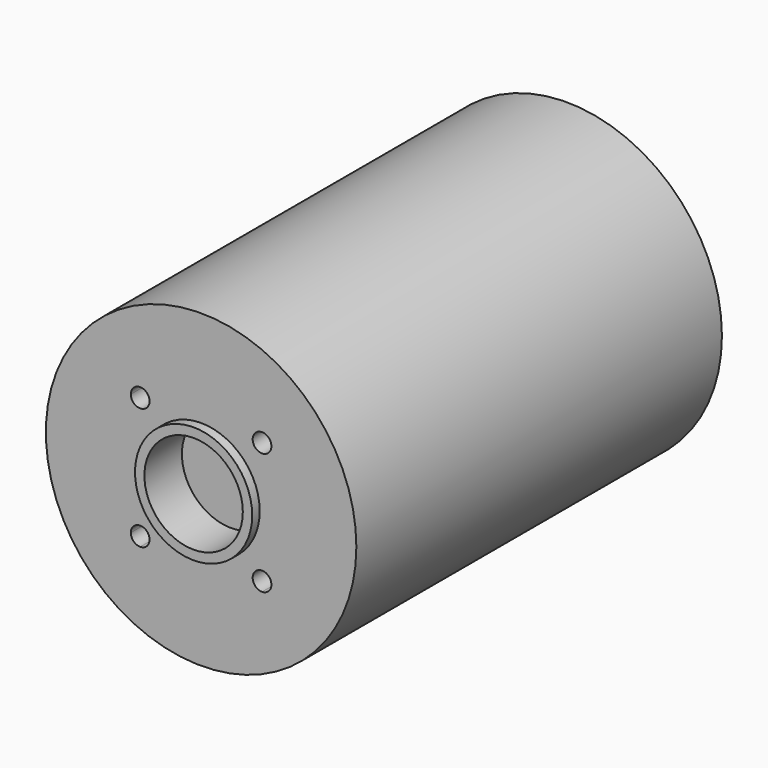
from build123d import *

# Parameters (mm, degrees)
F0_R     = 84.1375
F1_DEPTH = 247.65
F2_R     = 31.75
F3_DEPTH = 5.08
F5_DEPTH = 25.4
F6_R     = 26.67
F7_DEPTH = 25.4


# Not quite as in the source:
# - a feature names something its author has since deleted; it is built from what else it names


with BuildPart() as f1:
    # F0 (on Front) → F1 (new body)
    with BuildSketch(Plane.XZ):
        Circle(F0_R)
    extrude(amount=F1_DEPTH)

    # F2 (on face) → F3 (join)
    with BuildSketch(Plane.XZ.offset(247.65)):
        Circle(F2_R)
    extrude(amount=F3_DEPTH)

    # F4 (on face) → F5 (cut)
    with BuildSketch(Plane.XZ.offset(247.65)):
        with BuildLine():
            ThreePointArc((-27.94, 33.02), (-29.4278975516, 36.6121024484), (-33.02, 38.1))
            ThreePointArc((-33.02, 38.1), (-36.6121024484, 36.6121024484), (-38.1, 33.02))
            ThreePointArc((-38.1, 33.02), (-33.02, 27.94), (-27.94, 33.02))
        make_face()
        with BuildLine():
            ThreePointArc((38.1, 33.02), (36.6121024484, 36.6121024484), (33.02, 38.1))
            ThreePointArc((33.02, 38.1), (29.4278975516, 29.4278975516), (38.1, 33.02))
        make_face()
        with BuildLine():
            ThreePointArc((33.02, -38.1), (36.6121024484, -36.6121024484), (38.1, -33.02))
            ThreePointArc((38.1, -33.02), (29.4278975516, -29.4278975516), (33.02, -38.1))
        make_face()
        with BuildLine():
            ThreePointArc((-27.94, -33.02), (-33.02, -27.94), (-38.1, -33.02))
            ThreePointArc((-38.1, -33.02), (-36.6121024484, -36.6121024484), (-33.02, -38.1))
            ThreePointArc((-33.02, -38.1), (-29.4278975516, -36.6121024484), (-27.94, -33.02))
        make_face()
    extrude(amount=-F5_DEPTH, mode=Mode.SUBTRACT)

    # F6 (on face) → F7 (cut)
    with BuildSketch(Plane.XZ.offset(252.73)):
        Circle(F6_R)
    extrude(amount=-F7_DEPTH, mode=Mode.SUBTRACT)


solid = f1.part
